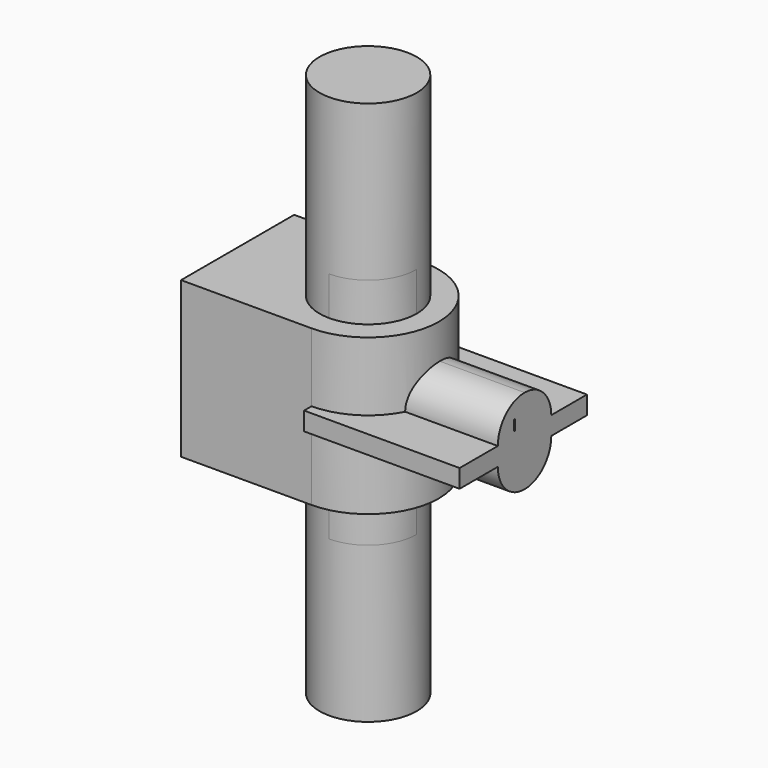
from build123d import *

# Parameters (mm, degrees)
F1_DEPTH   = 110
F1_FACE_R  = 27.5
F1_FACE1_R = 27.5
F3_DEPTH   = 44
F2_W       = 27.013732
F2_H       = 10.355262
F2_W_2     = 0.674465
F2_H_2     = 5.803441
F2_W_3     = 25.212824
F4_DEPTH   = 88


with BuildPart() as f1:
    # F0 (on Top) → F1 (new body, symmetric)
    with BuildSketch(Plane.XY):
        with BuildLine():
            ThreePointArc((27.5, 31.783064), (19.445436, 51.228501), (0, 59.283064))
            Line((0, 59.283064), (0, 4.283064))
            ThreePointArc((0, 4.283064), (19.445436, 12.337628), (27.5, 31.783064))
        make_face()
        with BuildLine():
            Line((0, 4.283064), (0, 59.283064))
            ThreePointArc((0, 59.283064), (-27.5, 31.783064), (0, 4.283064))
        make_face()
    extrude(amount=F1_DEPTH, both=True)

    # F0 (on Top) + F1_face (on face) + F1_face1 (on face) → F3 (join, symmetric)
    with BuildSketch(Plane.XY):
        with BuildLine():
            Line((0, 71.783064), (-73.839367, 71.783064))
            Line((-73.839367, 71.783064), (-73.839367, -8.216936))
            Line((-73.839367, -8.216936), (0, -8.216936))
            Line((0, -8.216936), (0, 4.283064))
            ThreePointArc((0, 4.283064), (-27.5, 31.783064), (0, 59.283064))
            Line((0, 59.283064), (0, 71.783064))
        make_face()
        with BuildLine():
            ThreePointArc((0, -8.216936), (40, 31.783064), (0, 71.783064))
            Line((0, 71.783064), (0, 59.283064))
            ThreePointArc((0, 59.283064), (19.445436, 51.228501), (27.5, 31.783064))
            ThreePointArc((27.5, 31.783064), (19.445436, 12.337628), (0, 4.283064))
            Line((0, 4.283064), (0, -8.216936))
        make_face()
    with BuildSketch(Plane(origin=(0, 31.783064, -110), x_dir=(1, 0, 0), z_dir=(0, 0, -1))):
        Circle(F1_FACE_R)
    with BuildSketch(Plane(origin=(0, 31.783064, 110), x_dir=(1, 0, 0), z_dir=(0, 0, 1))):
        Circle(F1_FACE1_R)
    extrude(amount=F3_DEPTH, both=True, dir=(0, 0, 1))

    # F2 (on Right) → F4 (join)
    with BuildSketch(Plane.YZ):
        Rectangle(F2_W, F2_H)
        with BuildLine():
            ThreePointArc((32.416481, 24.087246), (19.045364, 18.548748), (13.506866, 5.177631))
            Line((13.506866, 5.177631), (13.506866, -5.177631))
            ThreePointArc((13.506866, -5.177631), (24.488906, -2.78886), (32.416481, 5.177631))
            ThreePointArc((32.416481, 5.177631), (30.021819, 14.632438), (32.416481, 24.087246))
        make_face()
        with Locations((25.447267, 10.780724)):
            Rectangle(F2_W_2, F2_H_2, mode=Mode.SUBTRACT)
        with BuildLine():
            ThreePointArc((32.416481, 5.177631), (24.488906, -2.78886), (13.506866, -5.177631))
            ThreePointArc((13.506866, -5.177631), (32.416481, -24.087246), (51.326096, -5.177631))
            ThreePointArc((51.326096, -5.177631), (40.344056, -2.78886), (32.416481, 5.177631))
        make_face()
        with BuildLine():
            ThreePointArc((51.326096, 5.177631), (45.787598, 18.548748), (32.416481, 24.087246))
            ThreePointArc((32.416481, 24.087246), (34.811143, 14.632438), (32.416481, 5.177631))
            ThreePointArc((32.416481, 5.177631), (40.344056, -2.78886), (51.326096, -5.177631))
            Line((51.326096, -5.177631), (51.326096, 5.177631))
        make_face()
        with BuildLine():
            ThreePointArc((32.416481, 5.177631), (34.811143, 14.632438), (32.416481, 24.087246))
            ThreePointArc((32.416481, 24.087246), (30.021819, 14.632438), (32.416481, 5.177631))
        make_face()
        with Locations((63.932508, 0)):
            Rectangle(F2_W_3, F2_H)
    extrude(amount=F4_DEPTH)


solid = f1.part
